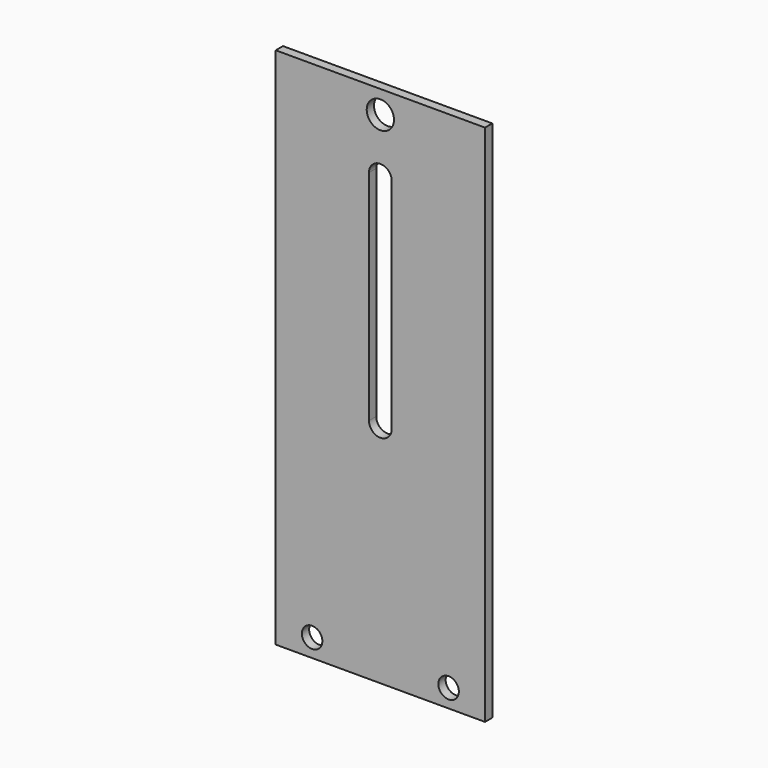
from build123d import *

# Parameters (mm, degrees)
F0_W     = 92
F0_H     = 230
F1_DEPTH = 4
F3_D     = 9
F4_D     = 12
F6_DEPTH = 4


with BuildPart() as f1:
    # F0 (on Front) → F1 (new body)
    with BuildSketch(Plane.XZ):
        with Locations((46, 115)):
            Rectangle(F0_W, F0_H)
    extrude(amount=F1_DEPTH)

    # F3 (through all)
    with Locations(Plane.XZ.offset(4)):
        with Locations((16, 8), (76, 8)):
            Hole(F3_D / 2)

    # F4 (through all)
    with Locations(Plane.XZ.offset(4)):
        with Locations((46, 220)):
            Hole(F4_D / 2)

    # F5 (on face) → F6 (cut, through all)
    with BuildSketch(Plane.XZ.offset(4)):
        with BuildLine():
            ThreePointArc((41, 100), (46, 95), (51, 100))
            Line((51, 100), (51, 196))
            ThreePointArc((51, 196), (46, 201), (41, 196))
            Line((41, 196), (41, 100))
        make_face()
    extrude(amount=-F6_DEPTH, mode=Mode.SUBTRACT)


solid = f1.part
